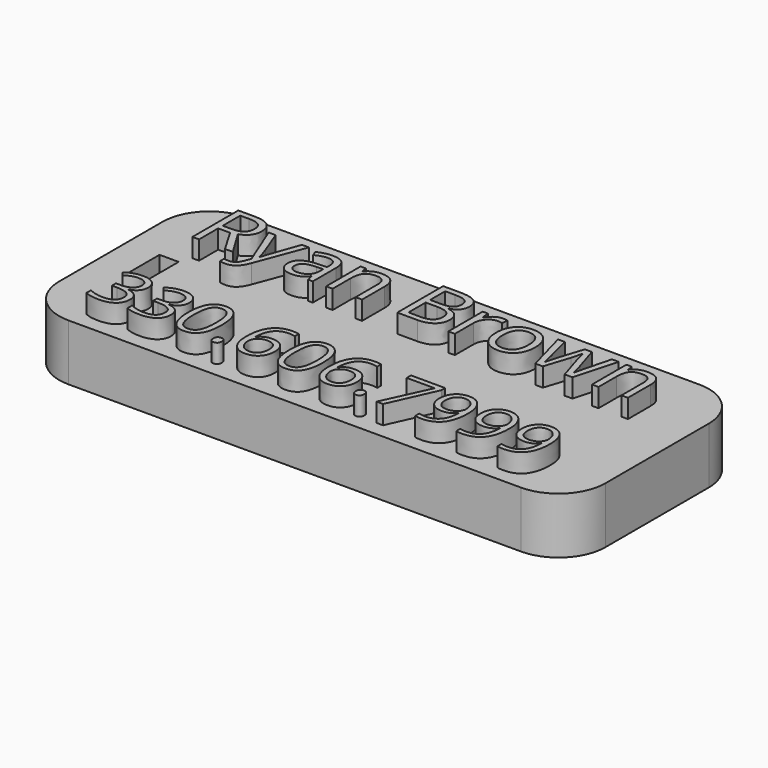
from build123d import *

# Parameters (mm, degrees)
F0_W         = 58.2218244672
F0_H         = 23.7748990767
F1_DEPTH     = 6
F2_R         = 5
F5_TEXT_SIZE = 7.6669661575
F4_TEXT_SIZE = 8.5560171606
F6_DEPTH     = 2
F7_W         = 2.0408891141
F7_H         = 4.1555203497
F8_DEPTH     = 6


# Not quite as in the source:
# - Text() gives the source's letters only with a copy of the font that has no kerning and outlines rounded to 1/6400 em; it was checked with that copy


with BuildPart() as f1:
    # F0 (on Top) → F1 (new body)
    with BuildSketch(Plane.XY):
        Rectangle(F0_W, F0_H)
    extrude(amount=F1_DEPTH)

    # F2
    f2_edges = [f1.edges().sort_by_distance(p)[0] for p in [
        (-29.110912, 11.88745, 3),
        (29.110912, 11.88745, 3),
        (29.110912, -11.88745, 3),
        (-29.110912, -11.88745, 3),
    ]]
    fillet(f2_edges, radius=F2_R)

    # F5 (on face) + F4 (on face) → F6 (join)
    with BuildSketch(Plane.XY.offset(6)):
        with Locations((-24, -10.2930826266)):
            Text('330.606.7999', F5_TEXT_SIZE, font='Open Sans', text_align=(TextAlign.LEFT, TextAlign.BOTTOM))
    with BuildSketch(Plane.XY.offset(6)):
        with Locations((-23.905378259, 3.3106910996)):
            Text('Ryan Brown', F4_TEXT_SIZE, font='Open Sans', text_align=(TextAlign.LEFT, TextAlign.BOTTOM))
    extrude(amount=F6_DEPTH)

    # F7 (on face) → F8 (cut, through all)
    with BuildSketch(Plane.XY.offset(6)):
        with Locations((-24.5690140873, 0)):
            Rectangle(F7_W, F7_H)
    extrude(amount=-F8_DEPTH, mode=Mode.SUBTRACT)


solid = f1.part
